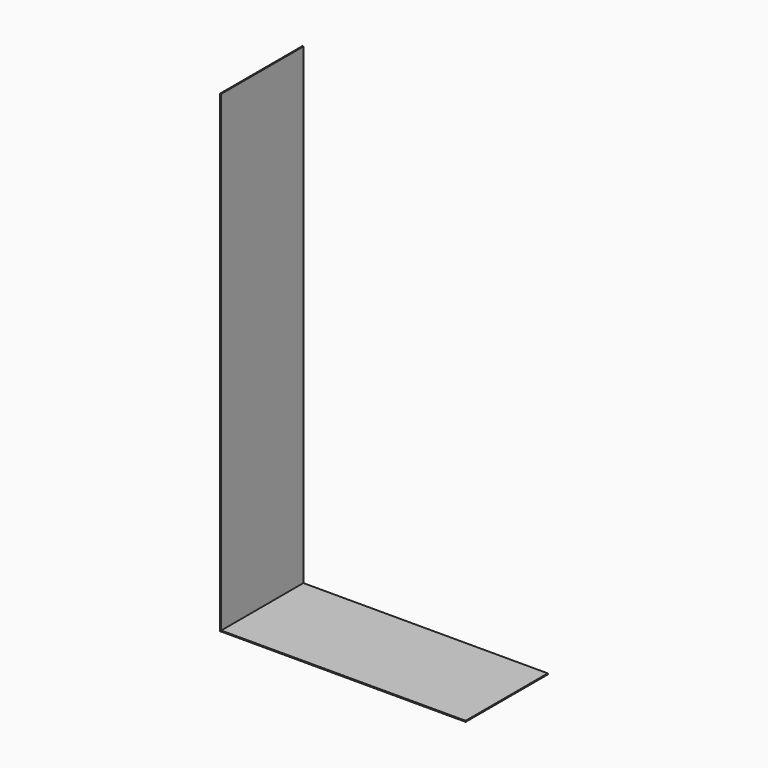
from build123d import *

# Parameters (mm, degrees)
F0_W     = 1190
F0_H     = 500
F1_DEPTH = 5
F2_W     = 500
F2_H     = 5
F2_H_2   = 2300
F3_DEPTH = 5


# Not quite as in the source:
# - the program builds the solid bodies; features that only make, move or delete a surface that nothing else refers to are left out


with BuildPart() as f1:
    # F0 (on Top) → F1 (new body)
    with BuildSketch(Plane.XY):
        Rectangle(F0_W, F0_H)
    extrude(amount=-F1_DEPTH)

    # F2 (on face) → F3 (join)
    with BuildSketch(Plane(origin=(-595, 0, 0), x_dir=(0, -1, 0), z_dir=(-1, 0, 0))):
        with Locations((0, -2.5)):
            Rectangle(F2_W, F2_H)
        with Locations((0, 1150)):
            Rectangle(F2_W, F2_H_2)
    extrude(amount=F3_DEPTH)


solid = f1.part
